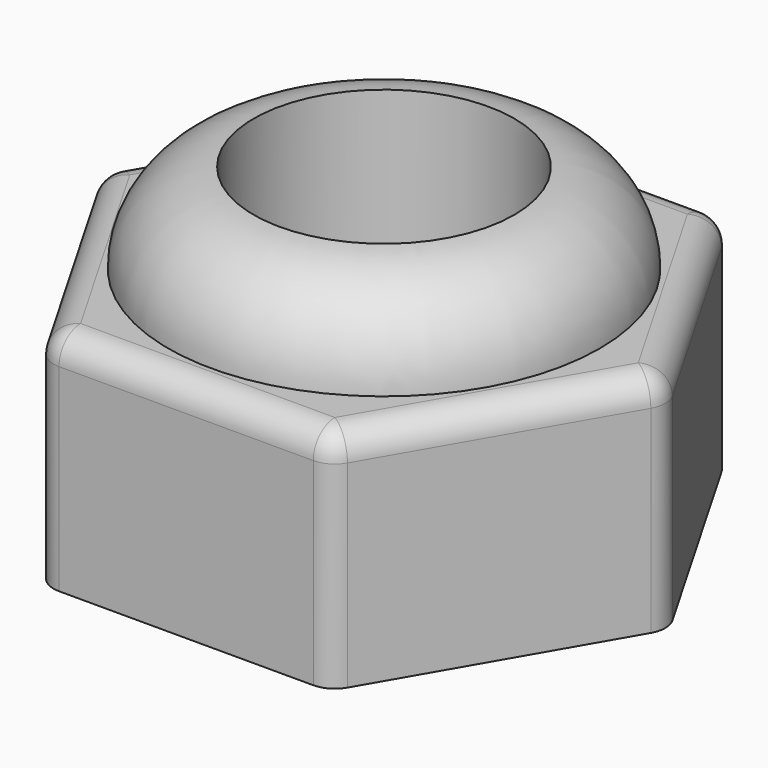
from build123d import *

# Parameters (mm, degrees)
F0_R     = 1.45
F1_DEPTH = 2.5
F3_R     = 2.4
F3_R_2   = 1.45
F4_DEPTH = 1
F5_R     = 0.3


# Not quite as in the source:
# - a fillet or chamfer that OpenCascade refuses, or shapes differently, is made with other operations: its cross-section is extruded or revolved along the edge and cut away or added


with BuildPart() as f1:
    # F0 (on Top) → F1 (new body)
    with BuildSketch(Plane.XY):
        Polygon((-1.5886400056, -2.7494647235), (1.5867862946, -2.7505349641), (3.1754263002, -0.0010702406), (1.5886400056, 2.7494647235), (-1.5867862946, 2.7505349641), (-3.1754263002, 0.0010702406), align=None)
        Circle(F0_R, mode=Mode.SUBTRACT)
    extrude(amount=F1_DEPTH)

    # F3 (on offset) → F4 (join)
    with BuildSketch(Plane.XY.offset(2.5)):
        Circle(F3_R)
        Circle(F3_R_2, mode=Mode.SUBTRACT)
    extrude(amount=F4_DEPTH)

    # F5
    f5_edges = [f1.edges().sort_by_distance(p)[0] for p in [
        (-2.382033, -1.374197, 2.5),
        (-2.381106, 1.375803, 2.5),
        (0.000927, 2.75, 2.5),
        (2.382033, 1.374197, 2.5),
        (2.381106, -1.375803, 2.5),
        (-0.000927, -2.75, 2.5),
        (3.175426, -0.00107, 1.25),
        (1.58864, 2.749465, 1.25),
        (-1.586786, 2.750535, 1.25),
        (-3.175426, 0.00107, 1.25),
        (-1.58864, -2.749465, 1.25),
        (1.586786, -2.750535, 1.25),
    ]]
    fillet(f5_edges, radius=F5_R)

    # F6: fillet of radius 1 on 1 edges, made by hand

    # F6_s1 → F6_t2 (revolve, cut)
    with BuildSketch(Plane.XZ):
        with BuildLine():
            ThreePointArc((1.45, 3.5), (2.1245688373, 3.1904532198), (2.4, 2.5012507822))
            Line((2.4, 2.5012507822), (2.4, 3.5))
            Line((2.4, 3.5), (1.45, 3.5))
        make_face()
    revolve(axis=Axis((0, 0, 3.5), (0, 0, 1)), mode=Mode.SUBTRACT)


solid = f1.part
